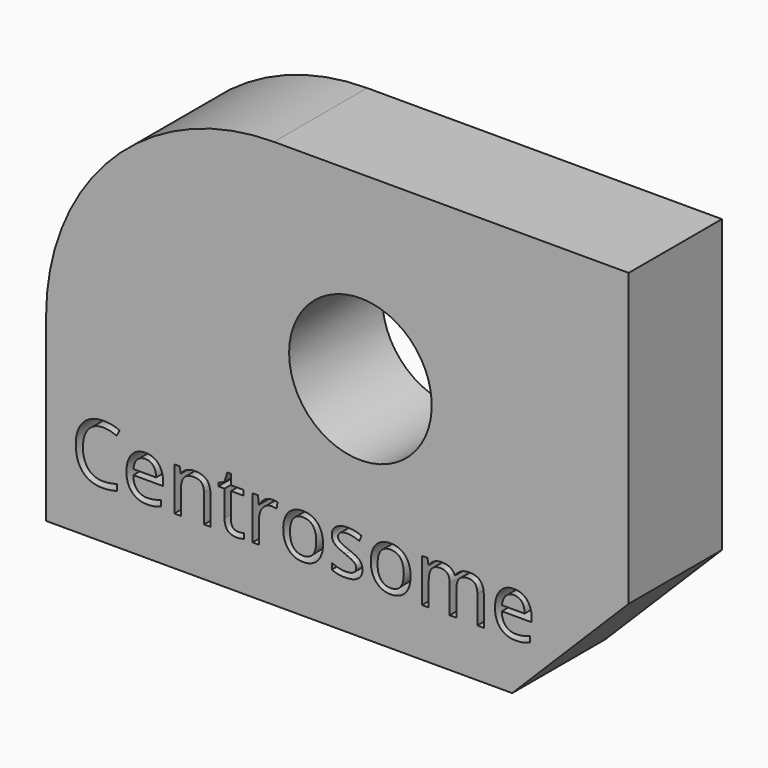
from build123d import *

# Parameters (mm, degrees)
F0_W         = 127
F0_H         = 88.9
F1_DEPTH     = 25.4
F2_R         = 49.6700298323
F3_SIZE      = 25.4
F4_R         = 15.5467172279
F5_DEPTH     = 38.1
F6_TEXT_SIZE = 17.651338292
F7_DEPTH     = 14.732


# Not quite as in the source:
# - Text() gives the source's letters only with a copy of the font that has no kerning and outlines rounded to 1/6400 em; it was checked with that copy


with BuildPart() as f1:
    # F0 (on Front) → F1 (new body)
    with BuildSketch(Plane.XZ):
        with Locations((0.988714397, -5.0414916958)):
            Rectangle(F0_W, F0_H)
    extrude(amount=F1_DEPTH)

    # F2
    f2_edges = [f1.edges().sort_by_distance(p)[0] for p in [
        (-62.511286, -12.7, 39.408508),
    ]]
    fillet(f2_edges, radius=F2_R)

    # F3
    f3_edges = [f1.edges().sort_by_distance(p)[0] for p in [
        (64.488714, -12.7, -49.491492),
    ]]
    chamfer(f3_edges, length=F3_SIZE)

    # F4 (on face) → F5 (cut)
    with BuildSketch(Plane(origin=(0, 0, 0), x_dir=(-1, 0, 0), z_dir=(0, 1, 0))):
        with Locations((-6.0083568096, 0)):
            Circle(F4_R)
    extrude(amount=-F5_DEPTH, mode=Mode.SUBTRACT)

    # F6 (on face) → F7 (cut)
    with BuildSketch(Plane.XZ.offset(25.4)):
        with Locations((-57.1224911378, -38.978383497)):
            Text('Centrosome', F6_TEXT_SIZE, font='Open Sans', text_align=(TextAlign.LEFT, TextAlign.BOTTOM))
    extrude(amount=-F7_DEPTH, mode=Mode.SUBTRACT)


solid = f1.part
